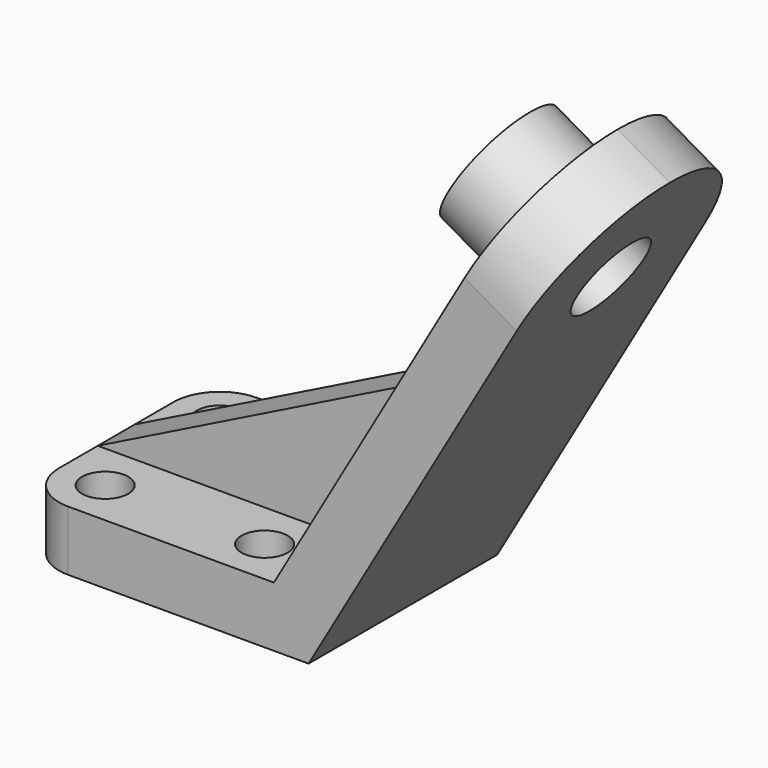
from build123d import *

# Parameters (mm, degrees)
F1_DEPTH  = 102
F2_R      = 50.99999
F3_R      = 27
F3_R_2    = 18.5
F4_DEPTH  = 30
F5_R      = 18.5
F6_DEPTH  = 30
F9_DEPTH  = 10
F10_R     = 10
F11_DEPTH = 30
F12_R     = 20


# Not quite as in the source:
# - a fillet or chamfer is up to 0.001 mm smaller than in the source, because OpenCascade refuses the exact size


with BuildPart() as f1:
    # F0 (on Front) → F1 (new body)
    with BuildSketch(Plane.XZ):
        Polygon((-15.0111069989, -63.9414438152), (-124.0111069989, -63.9414438152), (-124.0111069989, -89.9414438152), (0, -89.9414438152), (115.5, 110.110424459), (92.9833395016, 123.110424459), align=None)
    extrude(amount=F1_DEPTH)

    # F2 (radius 51 in the source; OpenCascade refuses exactly that, so slightly less here)
    f2_edges = [f1.edges().sort_by_distance(p)[0] for p in [
        (104.24167, 0, 116.610424),
        (104.24167, -102, 116.610424),
    ]]
    fillet(f2_edges, radius=F2_R)

    # F3 (on face) → F4 (join)
    with BuildSketch(Plane(origin=(16.4291271001, 0, -9.4853609538), x_dir=(0, -1, 0), z_dir=(-0.8660254038, 0, 0.5))):
        with Locations((51, 102.108424803)):
            Circle(F3_R)
        with Locations((51, 102.108424803)):
            Circle(F3_R_2, mode=Mode.SUBTRACT)
    extrude(amount=F4_DEPTH)

    # F5 (on face) → F6 (cut)
    with BuildSketch(Plane(origin=(16.4291271001, 0, -9.4853609538), x_dir=(0, -1, 0), z_dir=(-0.8660254038, 0, 0.5))):
        with Locations((51, 102.108424803)):
            Circle(F5_R)
    extrude(amount=-F6_DEPTH, mode=Mode.SUBTRACT)

    # F8 (on offset) → F9 (join, symmetric)
    with BuildSketch(Plane(origin=(0, -51, 0), x_dir=(-1, 0, 0), z_dir=(0, 1, 0))):
        Polygon((-28.8675134595, 12.0585561848), (15.0111069989, -63.9414438152), (124.0111069989, -63.9414438152), align=None)
    extrude(amount=F9_DEPTH, both=True)

    # F10 (on face) → F11 (cut)
    with BuildSketch(Plane.XY.offset(-63.9414438152)):
        with Locations((-104.0111069989, -20)):
            Circle(F10_R)
        with Locations((-104.0111069989, -82)):
            Circle(F10_R)
        with Locations((-35.0111069989, -20)):
            Circle(F10_R)
        with Locations((-35.0111069989, -82)):
            Circle(F10_R)
    extrude(amount=-F11_DEPTH, mode=Mode.SUBTRACT)

    # F12
    f12_edges = [f1.edges().sort_by_distance(p)[0] for p in [
        (-124.011107, 0, -76.941444),
        (-124.011107, -102, -76.941444),
    ]]
    fillet(f12_edges, radius=F12_R)


solid = f1.part
